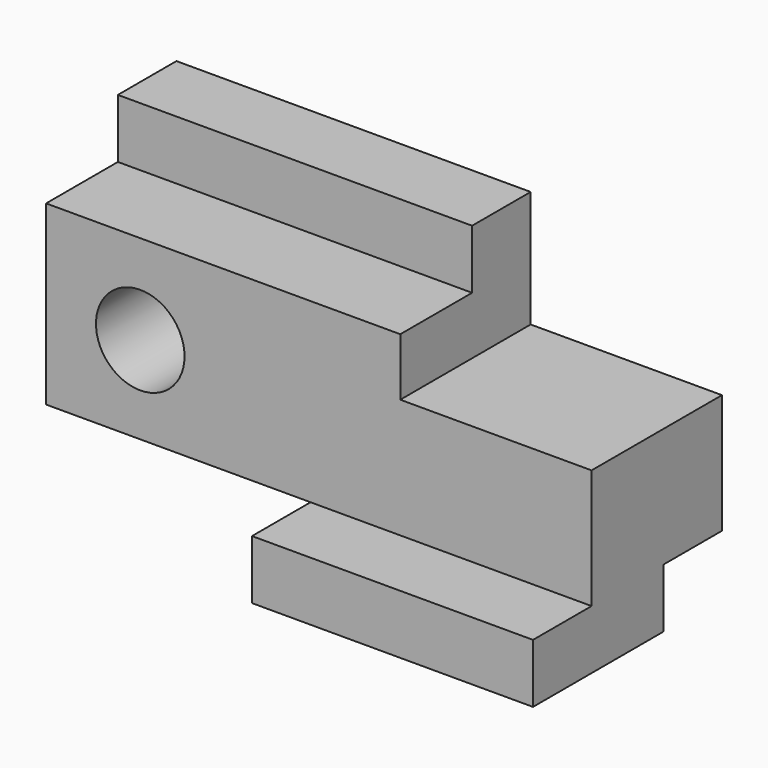
from build123d import *

# Parameters (mm, degrees)
F0_W      = 117.348
F0_H      = 63.5
F1_DEPTH  = 50.8
F2_W      = 35.052
F2_H      = 12.7
F3_DEPTH  = 117.349
F4_W      = 15.748
F4_H      = 38.1
F5_DEPTH  = 207
F6_DEPTH  = 117.349
F7_W      = 41.148
F7_H      = 25.4409682324
F8_DEPTH  = 35.053
F9_W      = 56.896
F9_H      = 12.7
F10_DEPTH = 50.801
F11_W     = 15.748
F11_H     = 12.7
F12_DEPTH = 117.349
F13_R     = 9.525
F14_DEPTH = 35.053


# Not quite as in the source:
# - an extrude ends at something that could not be found from the text; its depth is read off the source's solid


with BuildPart() as f1:
    # F0 (on Front) → F1 (new body)
    with BuildSketch(Plane.XZ):
        Rectangle(F0_W, F0_H)
    extrude(amount=F1_DEPTH)

    # F2 (on face) → F3 (cut, through all)
    with BuildSketch(Plane(origin=(-58.674, 0, 0), x_dir=(0, -1, 0), z_dir=(-1, 0, 0))):
        with Locations((33.274, 25.4)):
            Rectangle(F2_W, F2_H)
    extrude(amount=-F3_DEPTH, mode=Mode.SUBTRACT)

    # F4 (on face) → F5 (cut, through all)
    with BuildSketch(Plane.YZ.offset(58.674)):
        with Locations((-42.926, 0)):
            Rectangle(F4_W, F4_H)
    extrude(amount=F5_DEPTH, mode=Mode.SUBTRACT)

    # F4 (on face) → F6 (cut, through all)
    with BuildSketch(Plane.YZ.offset(58.674)):
        with Locations((-42.926, 0)):
            Rectangle(F4_W, F4_H)
    extrude(amount=-F6_DEPTH, mode=Mode.SUBTRACT)

    # F7 (on face) → F8 (cut, through all)
    with BuildSketch(Plane.XZ.offset(35.052)):
        with Locations((38.1, 19.3680736702)):
            Rectangle(F7_W, F7_H)
    extrude(amount=-F8_DEPTH, mode=Mode.SUBTRACT)

    # F9 (on face) → F10 (cut, through all)
    with BuildSketch(Plane.XZ.offset(50.8)):
        with Locations((-30.226, -25.4)):
            Rectangle(F9_W, F9_H)
    extrude(amount=-F10_DEPTH, mode=Mode.SUBTRACT)

    # F11 (on face) → F12 (cut, through all)
    with BuildSketch(Plane.YZ.offset(58.674)):
        with Locations((-7.874, -25.4)):
            Rectangle(F11_W, F11_H)
    extrude(amount=-F12_DEPTH, mode=Mode.SUBTRACT)

    # F13 (on face) → F14 (cut, through all)
    with BuildSketch(Plane.XZ.offset(35.052)):
        with Locations((-38.413323462, -0.254)):
            Circle(F13_R)
    extrude(amount=-F14_DEPTH, mode=Mode.SUBTRACT)


solid = f1.part
